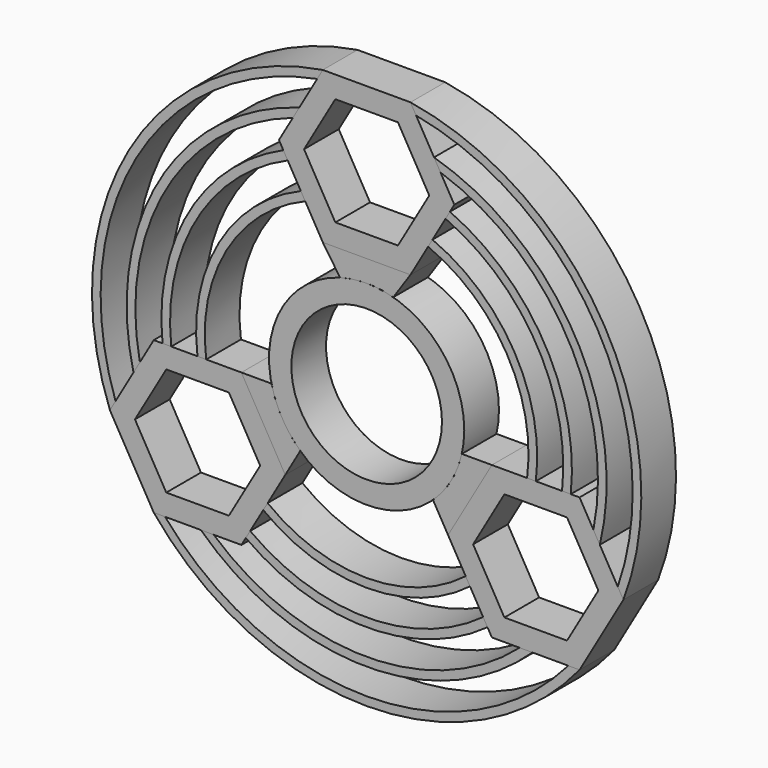
from build123d import *

# Parameters (mm, degrees)
F0_R     = 14.2875
F0_R_2   = 11.0236
F2_DEPTH = 6.35


# Not quite as in the source:
# - ends of sketch curves that miss each other by under 0.0002 mm in the source are joined


with BuildPart() as f2:
    # F0 (on Front) → F2 (new body)
    with BuildSketch(Plane.XZ):
        Circle(F0_R)
        Circle(F0_R_2, mode=Mode.SUBTRACT)
    extrude(amount=F2_DEPTH)


with BuildPart() as f2b:
    # F0 (on Front) → F2, piece 2 (new body)
    with BuildSketch(Plane.XZ):
        Polygon((-6.4158048664, 17.4625), (6.4158048664, 17.4625), (12.8316097327, 28.575), (6.4158048664, 39.6875), (-6.4158048664, 39.6875), (-12.8316097327, 28.575), align=None)
        Polygon((9.1654355234, 28.575), (4.5827177617, 20.6375), (-4.5827177617, 20.6375), (-9.1654355234, 28.575), (-4.5827177617, 36.5125), (4.5827177617, 36.5125), align=None, mode=Mode.SUBTRACT)
    extrude(amount=F2_DEPTH)


with BuildPart() as f2c:
    # F0 (on Front) → F2, piece 3 (new body)
    with BuildSketch(Plane.XZ):
        Polygon((-31.1624807795, -25.4), (-18.3308710468, -25.4), (-11.9150661804, -14.2875), (-18.3308710468, -3.175), (-31.1624807795, -3.175), (-37.5782856459, -14.2875), align=None)
        Polygon((-33.9121114365, -14.2875), (-29.3293936748, -6.35), (-20.1639581514, -6.35), (-15.5812403898, -14.2875), (-20.1639581514, -22.225), (-29.3293936748, -22.225), align=None, mode=Mode.SUBTRACT)
    extrude(amount=F2_DEPTH)


with BuildPart() as f2d:
    # F0 (on Front) → F2, piece 4 (new body)
    with BuildSketch(Plane.XZ):
        Polygon((37.5782856459, -14.2875), (31.1624807795, -3.175), (18.3308710468, -3.175), (11.9150661804, -14.2875), (18.3308710468, -25.4), (31.1624807795, -25.4), align=None)
        Polygon((29.3293936748, -22.225), (20.1639581514, -22.225), (15.5812403898, -14.2875), (20.1639581514, -6.35), (29.3293936748, -6.35), (33.9121114365, -14.2875), align=None, mode=Mode.SUBTRACT)
    extrude(amount=F2_DEPTH)


with BuildPart() as f2e:
    # F1 (on Front) → F2, piece 5 (new body)
    with BuildSketch(Plane.XZ):
        with BuildLine():
            ThreePointArc((-36.7535982008, -12.8590994448), (-33.7214703776, 19.4691), (-7.2404923114, 38.2590994448))
            Line((-7.2404923114, 38.2590994448), (-6.4158048664, 39.6875))
            ThreePointArc((-6.4158048664, 39.6875), (-34.8165931166, 20.1013694082), (-37.5782856459, -14.2875))
            Line((-37.5782856459, -14.2875), (-36.7535982008, -12.8590994448))
        make_face()
    extrude(amount=F2_DEPTH)


with BuildPart() as f2f:
    # F1 (on Front) → F2, piece 6 (new body)
    with BuildSketch(Plane.XZ):
        with BuildLine():
            Line((-10.8030992669, 32.0884831905), (-9.8641309809, 33.7148239686))
            ThreePointArc((-9.8641309809, 33.7148239686), (-30.4219135892, 17.5641), (-34.1299595314, -8.3148239686))
            Line((-34.1299595314, -8.3148239686), (-33.1909912454, -6.6884831905))
            ThreePointArc((-33.1909912454, -6.6884831905), (-29.3220613264, 16.9291), (-10.8030992669, 32.0884831905))
        make_face()
    extrude(amount=F2_DEPTH)


with BuildPart() as f2g:
    # F1 (on Front) → F2, piece 7 (new body)
    with BuildSketch(Plane.XZ):
        with BuildLine():
            ThreePointArc((-9.6331085014, 23.0350652667), (-21.6230914657, 12.4841069647), (-24.7655079948, -3.175))
            Line((-24.7655079948, -3.175), (-23.4845493514, -3.175))
            ThreePointArc((-23.4845493514, -3.175), (-20.523243224, 11.8491), (-8.9926440187, 21.9257163348))
            Line((-8.9926440187, 21.9257163348), (-9.6331085014, 23.0350652667))
        make_face()
    extrude(amount=F2_DEPTH)


with BuildPart() as f2h:
    # F1 (on Front) → F2, piece 8 (new body)
    with BuildSketch(Plane.XZ):
        with BuildLine():
            ThreePointArc((-28.6025203477, -3.175), (-24.9226522752, 14.3891), (-11.5516295168, 26.3580092334))
            Line((-11.5516295168, 26.3580092334), (-12.1903634715, 27.4643288954))
            ThreePointArc((-12.1903634715, 27.4643288954), (-26.022504538, 15.0241), (-29.879988257, -3.175))
            Line((-29.879988257, -3.175), (-28.6025203477, -3.175))
        make_face()
    extrude(amount=F2_DEPTH)


with BuildPart() as f2i:
    # F1 (on Front) → F2, piece 9 (new body)
    with BuildSketch(Plane.XZ):
        with BuildLine():
            ThreePointArc((-15.132397448, -19.860049313), (-8.0421e-06, -24.9682), (15.1323846544, -19.8600590611))
            Line((15.1323846544, -19.8600590611), (14.4919053327, -18.7507163348))
            ThreePointArc((14.4919053327, -18.7507163348), (0, -23.6982), (-14.4919053327, -18.7507163348))
            Line((-14.4919053327, -18.7507163348), (-15.132397448, -19.860049313))
        make_face()
    extrude(amount=F2_DEPTH)


with BuildPart() as f2j:
    # F1 (on Front) → F2, piece 10 (new body)
    with BuildSketch(Plane.XZ):
        with BuildLine():
            Line((17.6896247855, -24.2893288954), (17.0508908309, -23.1830092334))
            ThreePointArc((17.0508908309, -23.1830092334), (0, -28.7782), (-17.0508908309, -23.1830092334))
            Line((-17.0508908309, -23.1830092334), (-17.6896247855, -24.2893288954))
            ThreePointArc((-17.6896247855, -24.2893288954), (0, -30.0482), (17.6896247855, -24.2893288954))
        make_face()
    extrude(amount=F2_DEPTH)


with BuildPart() as f2k:
    # F1 (on Front) → F2, piece 11 (new body)
    with BuildSketch(Plane.XZ):
        with BuildLine():
            Line((-29.5131058894, -25.4), (-31.1624807795, -25.4))
            ThreePointArc((-31.1624807795, -25.4), (0, -40.2027388163), (31.1624807795, -25.4))
            Line((31.1624807795, -25.4), (29.5131058894, -25.4))
            ThreePointArc((29.5131058894, -25.4), (0, -38.9382), (-29.5131058894, -25.4))
        make_face()
    extrude(amount=F2_DEPTH)


with BuildPart() as f2l:
    # F1 (on Front) → F2, piece 12 (new body)
    with BuildSketch(Plane.XZ):
        with BuildLine():
            Line((-22.3878919785, -25.4), (-24.2658285505, -25.4))
            ThreePointArc((-24.2658285505, -25.4), (0, -35.1282), (24.2658285505, -25.4))
            Line((24.2658285505, -25.4), (22.3878919785, -25.4))
            ThreePointArc((22.3878919785, -25.4), (0, -33.8582), (-22.3878919785, -25.4))
        make_face()
    extrude(amount=F2_DEPTH)


with BuildPart() as f2m:
    # F1 (on Front) → F2, piece 13 (new body)
    with BuildSketch(Plane.XZ):
        with BuildLine():
            Line((9.6331233404, 23.0350590611), (8.9926440187, 21.9257163348))
            ThreePointArc((8.9926440187, 21.9257163348), (20.523243224, 11.8491), (23.4845493514, -3.175))
            Line((23.4845493514, -3.175), (24.7655059495, -3.175))
            ThreePointArc((24.7655059495, -3.175), (21.6230995078, 12.4840930353), (9.6331233404, 23.0350590611))
        make_face()
    extrude(amount=F2_DEPTH)


with BuildPart() as f2n:
    # F1 (on Front) → F2, piece 14 (new body)
    with BuildSketch(Plane.XZ):
        with BuildLine():
            Line((12.1903634715, 27.4643288954), (11.5516295168, 26.3580092334))
            ThreePointArc((11.5516295168, 26.3580092334), (24.9226522752, 14.3891), (28.6025203477, -3.175))
            Line((28.6025203477, -3.175), (29.879988257, -3.175))
            ThreePointArc((29.879988257, -3.175), (26.022504538, 15.0241), (12.1903634715, 27.4643288954))
        make_face()
    extrude(amount=F2_DEPTH)


with BuildPart() as f2o:
    # F1 (on Front) → F2, piece 15 (new body)
    with BuildSketch(Plane.XZ):
        with BuildLine():
            ThreePointArc((34.1299595314, -8.3148239686), (30.4219135892, 17.5641), (9.8641309809, 33.7148239686))
            Line((9.8641309809, 33.7148239686), (10.8030992669, 32.0884831905))
            ThreePointArc((10.8030992669, 32.0884831905), (29.3220613264, 16.9291), (33.1909912454, -6.6884831905))
            Line((33.1909912454, -6.6884831905), (34.1299595314, -8.3148239686))
        make_face()
    extrude(amount=F2_DEPTH)


with BuildPart() as f2p:
    # F1 (on Front) → F2, piece 16 (new body)
    with BuildSketch(Plane.XZ):
        with BuildLine():
            ThreePointArc((37.5782856459, -14.2875), (34.8165931166, 20.1013694082), (6.4158048664, 39.6875))
            Line((6.4158048664, 39.6875), (7.2404923114, 38.2590994448))
            ThreePointArc((7.2404923114, 38.2590994448), (33.7214703776, 19.4691), (36.7535982008, -12.8590994448))
            Line((36.7535982008, -12.8590994448), (37.5782856459, -14.2875))
        make_face()
    extrude(amount=F2_DEPTH)


with BuildPart() as f2q:
    # F1 (on Front) → F2, piece 17 (new body)
    with BuildSketch(Plane.XZ):
        with BuildLine():
            Line((15.1229684123, -8.7312503486), (18.3308710468, -3.175))
            Line((18.3308710468, -3.175), (13.930255965, -3.175))
            ThreePointArc((13.930255965, -3.175), (12.3733379566, -7.14375), (9.7147586395, -10.4764555469))
            Line((9.7147586395, -10.4764555469), (11.9150661804, -14.2875))
            Line((11.9150661804, -14.2875), (15.1229684123, -8.7312503486))
        make_face()
    extrude(amount=F2_DEPTH)


with BuildPart() as f2r:
    # F1 (on Front) → F2, piece 18 (new body)
    with BuildSketch(Plane.XZ):
        with BuildLine():
            Line((3.8920739769, 13.7471603034), (6.4158048664, 17.4625))
            Line((6.4158048664, 17.4625), (0, 17.4625))
            Line((0, 17.4625), (-6.4158048664, 17.4625))
            Line((-6.4158048664, 17.4625), (-3.8920739769, 13.7471603034))
            ThreePointArc((-3.8920739769, 13.7471603034), (0, 14.2875), (3.8920739769, 13.7471603034))
        make_face()
    extrude(amount=F2_DEPTH)


with BuildPart() as f2s:
    # F1 (on Front) → F2, piece 19 (new body)
    with BuildSketch(Plane.XZ):
        with BuildLine():
            ThreePointArc((-9.7147586395, -10.4764555469), (-12.3733379566, -7.14375), (-13.930255965, -3.175))
            Line((-13.930255965, -3.175), (-18.3308710468, -3.175))
            Line((-18.3308710468, -3.175), (-15.1229686466, -8.7312499429))
            Line((-15.1229686466, -8.7312499429), (-11.9150661804, -14.2875))
            Line((-11.9150661804, -14.2875), (-9.7147586395, -10.4764555469))
        make_face()
    extrude(amount=F2_DEPTH)


solid = Compound([f2.part, f2b.part, f2c.part, f2d.part, f2e.part, f2f.part, f2g.part, f2h.part, f2i.part, f2j.part, f2k.part, f2l.part, f2m.part, f2n.part, f2o.part, f2p.part, f2q.part, f2r.part, f2s.part])
